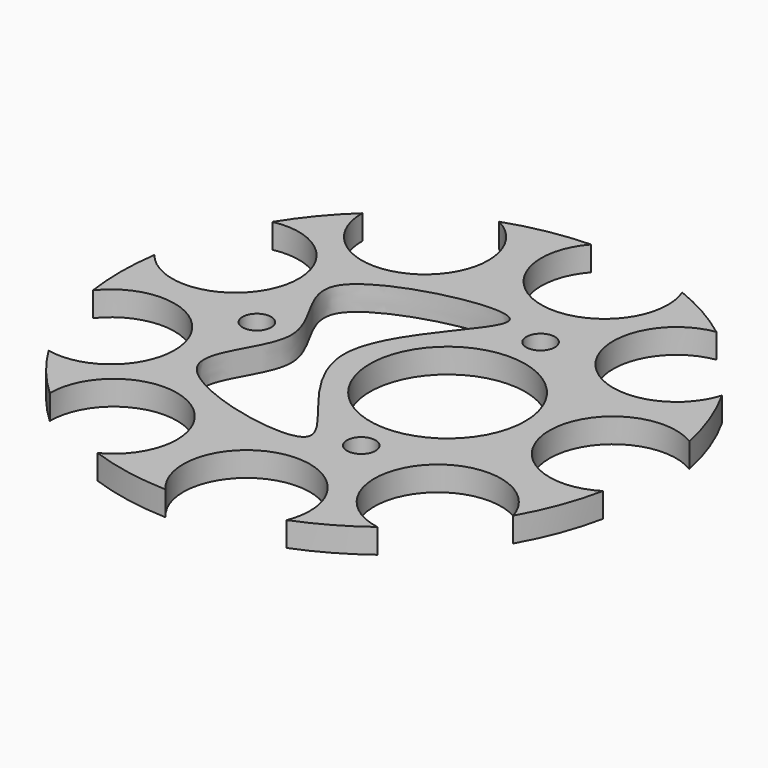
from build123d import *

# Parameters (mm, degrees)
F0_R     = 1.75
F0_R_2   = 9.5
F1_DEPTH = 3


with BuildPart() as f1:
    # F0 (on Top) → F1 (new body)
    with BuildSketch(Plane.XY):
        with BuildLine():
            ThreePointArc((31.8464317163, -6.633419719), (20.0305649598, -0.0256727641), (31.8633274362, 6.5517704478))
            ThreePointArc((31.8633274362, 6.5517704478), (30.4812860438, 11.3579740989), (28.3782402338, 15.8952453347))
            ThreePointArc((28.3782402338, 15.8952453347), (15.1284046954, 13.1169571507), (19.7307251041, 25.8486370824))
            ThreePointArc((19.7307251041, 25.8486370824), (16.0563808794, 28.274038207), (12.0879452, 30.1805780979))
            ThreePointArc((12.0879452, 30.1805780979), (12.4965108678, 28.7772522453), (12.6343334068, 27.3221734497))
            ThreePointArc((12.6343334068, 27.3221734497), (2.1202396518, 20.0818498579), (-0.8939983903, 32.4868013785))
            ThreePointArc((-0.8939983903, 32.4868013785), (-5.8671739777, 31.9603448058), (-10.7007039407, 30.6771378688))
            ThreePointArc((-10.7007039407, 30.6771378688), (-7.6366288229, 27.822401242), (-6.5051399496, 23.7903037152))
            ThreePointArc((-6.5051399496, 23.7903037152), (-14.304682236, 16.0404620677), (-22.0045065462, 23.8893862634))
            ThreePointArc((-22.0045065462, 23.8893862634), (-25.0311035566, 20.692030069), (-27.5977904465, 17.1149510223))
            ThreePointArc((-27.5977904465, 17.1149510223), (-21.1377458251, 15.5320899009), (-18.2837054482, 9.5244215205))
            ThreePointArc((-18.2837054482, 9.5244215205), (-23.4971338146, 2.2012866489), (-32.1232678605, 4.7307037955))
            ThreePointArc((-32.1232678605, 4.7307037955), (-32.469391937, 0.0416015456), (-32.1352863632, -4.6483723617))
            ThreePointArc((-32.1352863632, -4.6483723617), (-23.5120758979, -2.1378023923), (-18.3080294269, -9.4576808495))
            ThreePointArc((-18.3080294269, -9.4576808495), (-21.1697721423, -15.4716180556), (-27.6415625158, -17.0441769417))
            ThreePointArc((-27.6415625158, -17.0441769417), (-25.084051496, -20.62782222), (-22.0656587015, -23.8329245639))
            ThreePointArc((-22.0656587015, -23.8329245639), (-14.3556751017, -16.0038038715), (-6.5660636226, -23.7537026405))
            ThreePointArc((-6.5660636226, -23.7537026405), (-7.7027247217, -27.7942779191), (-10.7792890631, -30.6496235881))
            ThreePointArc((-10.7792890631, -30.6496235881), (-5.9490636133, -31.9452138205), (-0.9772535761, -32.4844140616))
            ThreePointArc((-0.9772535761, -32.4844140616), (2.0594816782, -20.0907523688), (12.5642953015, -27.3346119685))
            ThreePointArc((12.5642953015, -27.3346119685), (12.4246019524, -28.7994439311), (12.0105578361, -30.2114688529))
            ThreePointArc((12.0105578361, -30.2114688529), (15.9838666182, -28.3151056442), (19.6644146639, -25.8991291997))
            ThreePointArc((19.6644146639, -25.8991291997), (15.0947384847, -13.1556961205), (28.3374102331, -15.9679322398))
            ThreePointArc((28.3374102331, -15.9679322398), (30.4520773857, -11.4360656509), (31.8464317163, -6.633419719))
        make_face()
        with Locations((7.944258402, -13.7069351322)):
            Circle(F0_R, mode=Mode.SUBTRACT)
        with Locations((-15.7967726636, -4.44556e-05)):
            Circle(F0_R, mode=Mode.SUBTRACT)
        with BuildLine():
            add(Edge.make_bspline(
                [(-5.1607941213, -4.44556e-05), (-5.1607941213, 6.8016946043), (13.9227316309, 20.4717509816), (-22.4319309953, 12.4837041278), (-6.7623394337, -4.44556e-05), (-22.4319309953, -12.483793039), (13.9227316309, -20.4718398928), (-5.1607941213, -6.8017835155), (-5.1607941213, -4.44556e-05)],
                knots=[0, 0, 0, 0, 0.177937682, 0.3576170923, 0.5, 0.6423829077, 0.822062318, 1, 1, 1, 1], degree=3))
        make_face(mode=Mode.SUBTRACT)
        with Locations((7.5305884979, -0.0008045419)):
            Circle(F0_R_2, mode=Mode.SUBTRACT)
        with Locations((7.944258402, 13.7068462209)):
            Circle(F0_R, mode=Mode.SUBTRACT)
    extrude(amount=-F1_DEPTH)


solid = f1.part
